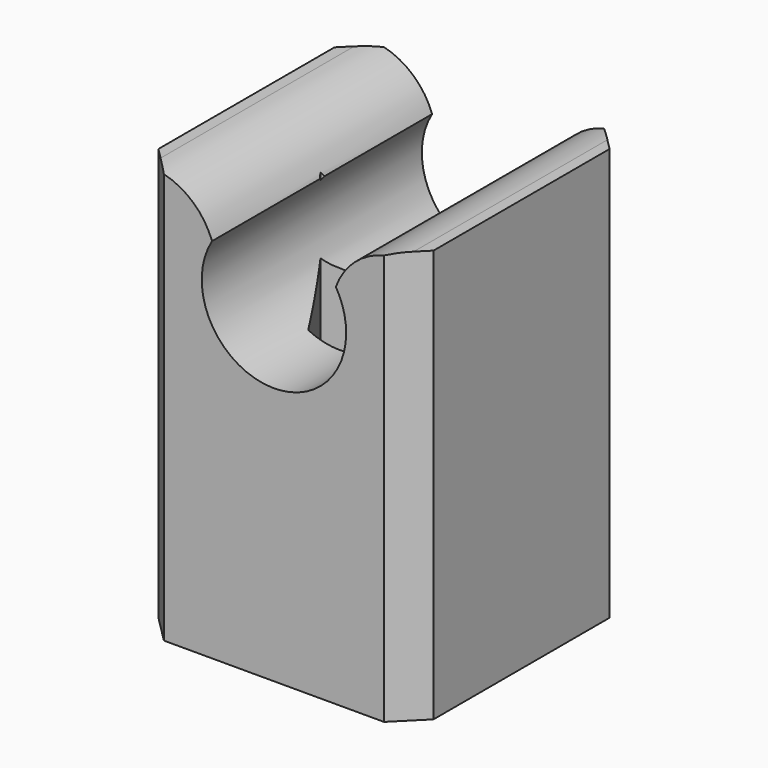
from build123d import *

# Parameters (mm, degrees)
F0_W        = 20
F0_H        = 20
F0_R        = 2.75
F1_DEPTH    = 15
F2_DEPTH    = 15
F4_DEPTH    = 20
F5_T1_DEPTH = 33.2973278516
F6_SIZE     = 2


# Not quite as in the source:
# - a fillet or chamfer that OpenCascade refuses, or shapes differently, is made with other operations: its cross-section is extruded or revolved along the edge and cut away or added


with BuildPart() as f1:
    # F0 (on Top) → F1 (new body)
    with BuildSketch(Plane.XY):
        Rectangle(F0_W, F0_H)
        Polygon((-4.6188021535, 0), (-2.3094010768, 4), (2.3094010768, 4), (4.6188021535, 0), (2.3094010768, -4), (-2.3094010768, -4), align=None, mode=Mode.SUBTRACT)
        Polygon((2.3094010768, 4), (-2.3094010768, 4), (-4.6188021535, 0), (-2.3094010768, -4), (2.3094010768, -4), (4.6188021535, 0), align=None)
        Circle(F0_R, mode=Mode.SUBTRACT)
    extrude(amount=-F1_DEPTH)

    # F0 (on Top) → F2 (join)
    with BuildSketch(Plane.XY):
        Rectangle(F0_W, F0_H)
        Polygon((-4.6188021535, 0), (-2.3094010768, 4), (2.3094010768, 4), (4.6188021535, 0), (2.3094010768, -4), (-2.3094010768, -4), align=None, mode=Mode.SUBTRACT)
    extrude(amount=F2_DEPTH)

    # F3 (on face) → F4 (cut, through all)
    with BuildSketch(Plane.XZ.offset(10)):
        with BuildLine():
            ThreePointArc((-4.5, 11.7041634566), (-1.40312152, 3.9409734138), (5.25, 9))
            ThreePointArc((5.25, 9), (5.0590265862, 10.40312152), (4.5, 11.7041634566))
            ThreePointArc((4.5, 11.7041634566), (0, 14.25), (-4.5, 11.7041634566))
        make_face()
        with BuildLine():
            ThreePointArc((-4.5, 11.7041634566), (0, 14.25), (4.5, 11.7041634566))
            Line((4.5, 11.7041634566), (4.5, 15))
            Line((4.5, 15), (-4.5, 15))
            Line((-4.5, 15), (-4.5, 11.7041634566))
        make_face()
    extrude(amount=-F4_DEPTH, mode=Mode.SUBTRACT)

    # F5: fillet of radius 5 on 2 edges, made by hand

    # F5_s2 → F5_t1 (cut)
    with BuildSketch(Plane.XZ.offset(-11.5457782428)):
        with BuildLine():
            ThreePointArc((-9.2006198435, 15), (-6.330151004, 14.0939478064), (-4.5, 11.7041634566))
            Line((-4.5, 11.7041634566), (-4.5, 15))
            Line((-4.5, 15), (-9.2006198435, 15))
        make_face()
        with BuildLine():
            ThreePointArc((9.2006198435, 15), (6.330151004, 14.0939478064), (4.5, 11.7041634566))
            Line((4.5, 11.7041634566), (4.5, 15))
            Line((4.5, 15), (9.2006198435, 15))
        make_face()
    extrude(amount=F5_T1_DEPTH, mode=Mode.SUBTRACT)

    # F6
    f6_edges = [f1.edges().sort_by_distance(p)[0] for p in [
        (-10, -10, 0),
        (10, -10, 0),
        (-10, 10, 0),
        (10, 10, 0),
    ]]
    chamfer(f6_edges, length=F6_SIZE)


solid = f1.part
